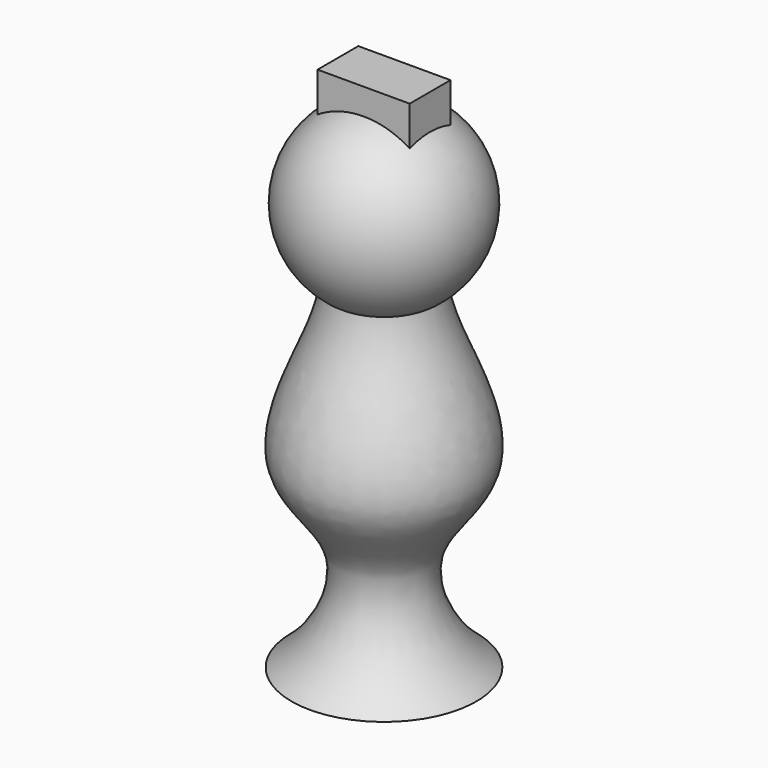
from build123d import *

# Parameters (mm, degrees)
F2_W     = 20.458
F2_H     = 11.3178063184
F3_DEPTH = 25
F10_T    = -2.5


# Not quite as in the source:
# - the program builds the solid bodies; features that only make, move or delete a surface that nothing else refers to are left out


with BuildPart() as f1:
    # F0 (on Front) → F1 (revolve)
    with BuildSketch(Plane.XZ):
        with BuildLine():
            Line((0, 20), (0, -20))
            ThreePointArc((0, -20), (20, 0), (0, 20))
        make_face()
    revolve(axis=Axis((0, 0, 0), (0, 0, -1)))

    # F2 (on Top) → F3 (join)
    with BuildSketch(Plane.XY):
        Rectangle(F2_W, F2_H)
    extrude(amount=F3_DEPTH)


with BuildPart() as f5:
    # F4 (on Front) → F5 (revolve)
    with BuildSketch(Plane.XZ):
        with BuildLine():
            Line((0, 0), (-13.7524965748, 0))
            add(Edge.make_bspline(
                [(-13.7524965748, 0), (-8.2117667219, -13.5443547456), (-15.7940470288, -29.097065496), (-24.5181266702, -52.895092497), (-4.983214771, -67.2633857979), (-12.2797935148, -84.0989501471), (-20.5344557762, -90.7746404409)],
                knots=[0, 0, 0, 0, 0.2850496582, 0.5219679881, 0.7448296737, 1, 1, 1, 1], degree=3))
            Line((-20.5344557762, -90.7746404409), (0, -90.7746404409))
            Line((0, -90.7746404409), (0, 0))
        make_face()
    revolve(axis=Axis((0, 0, -45.3873202205), (0, 0, -1)))

    # F10
    f10_openings = [f5.faces().sort_by_distance(p)[0] for p in [
        (0, 0, -90.77464),
    ]]
    offset(amount=F10_T, openings=f10_openings)


solid = Compound([f1.part, f5.part])
